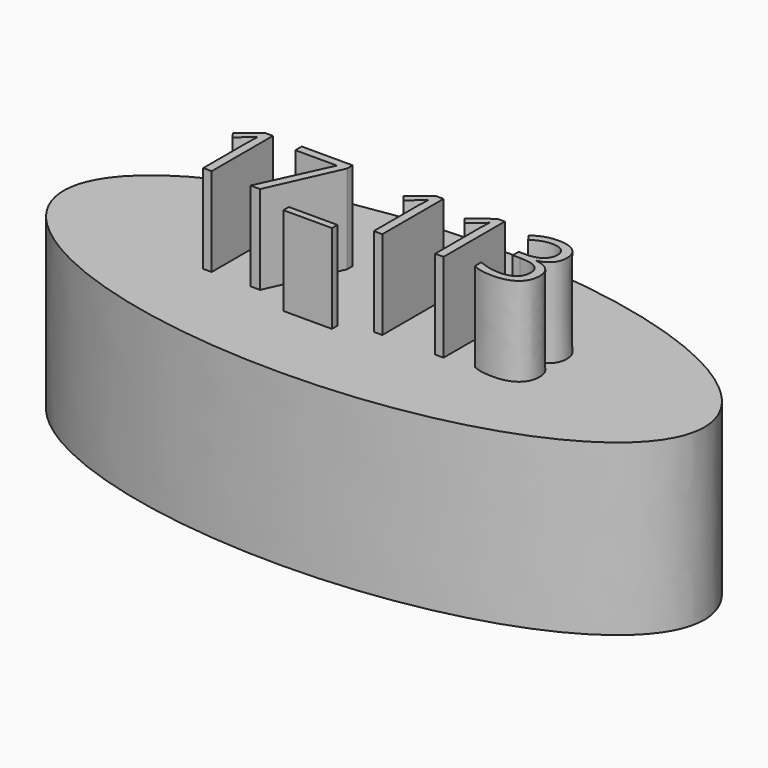
from build123d import *

# Parameters (mm, degrees)
F1_DEPTH     = 48.514
F2_TEXT_SIZE = 30.6659120921
F3_DEPTH     = 25.4


# Not quite as in the source:
# - Text() gives the source's letters only with a copy of the font that has no kerning and outlines rounded to 1/6400 em; it was checked with that copy


with BuildPart() as f1:
    # F0 (on Top) → F1 (new body)
    with BuildSketch(Plane.XY):
        with BuildLine():
            add(Edge.make_bspline(
                [(91.6459783912, 0), (91.6459783912, 66.677143268), (-45.8229891956, 33.338571634), (-183.2919567823, 0), (-45.8229891956, -33.338571634), (91.6459783912, -66.677143268), (91.6459783912, 0)],
                knots=[0, 0, 0, 2.0943951024, 2.0943951024, 4.1887902048, 4.1887902048, 6.2831853072, 6.2831853072, 6.2831853072], degree=2, weights=[1, 0.5, 1, 0.5, 1, 0.5, 1]))
        make_face()
    extrude(amount=F1_DEPTH)

    # F2 (on face) → F3 (join)
    with BuildSketch(Plane.XY.offset(48.514)):
        with Locations((-51.9132010127, -10.1151495613)):
            Text('17_113', F2_TEXT_SIZE, font='Open Sans', text_align=(TextAlign.LEFT, TextAlign.BOTTOM))
    extrude(amount=F3_DEPTH)


solid = f1.part
